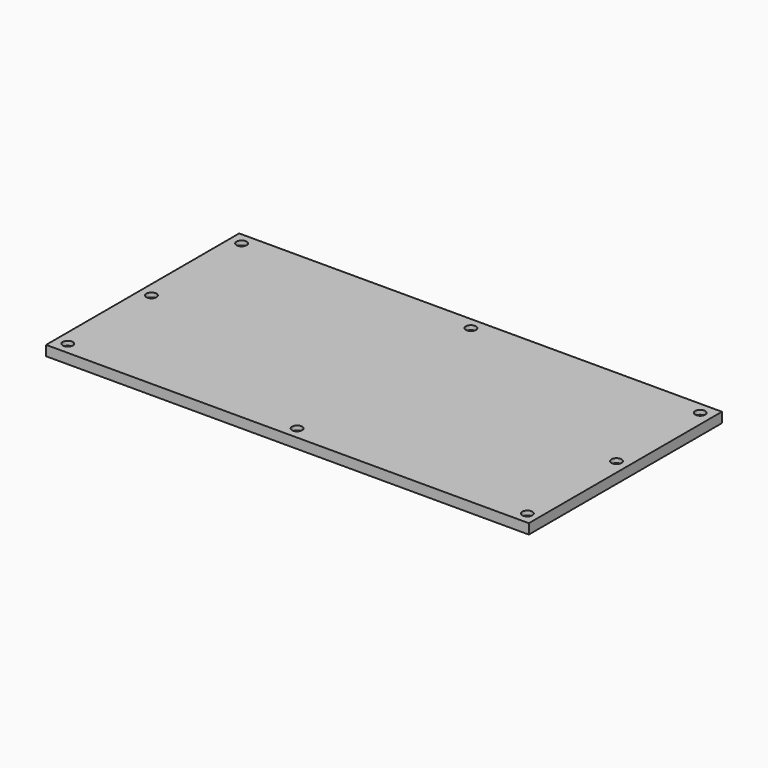
from build123d import *

# Parameters (mm, degrees)
F0_W           = 152.4
F0_H           = 76.2
F1_DEPTH       = 3.175
F3_D           = 3.175
F3_CSINK_D     = 6.35
F3_CSINK_ANGLE = 82


# Not quite as in the source:
# - a feature names something its author has since deleted; it is built from what else it names


with BuildPart() as f1:
    # F0 (on Top) → F1 (new body)
    with BuildSketch(Plane.XY):
        with Locations((76.2, 38.1)):
            Rectangle(F0_W, F0_H)
    extrude(amount=F1_DEPTH)

    # F3 (through all)
    with Locations(Plane(origin=(0, 0, 0), x_dir=(1, 0, 0), z_dir=(0, 0, -1))):
        with Locations((3.81, -3.81), (3.81, -36.83), (3.81, -72.39), (148.59, -72.39), (148.59, -39.37), (148.59, -457.2), (76.2, -3.81), (76.2, -72.39), (148.9000022411, -3.81)):
            CounterSinkHole(F3_D / 2, F3_CSINK_D / 2, counter_sink_angle=F3_CSINK_ANGLE)


solid = f1.part
